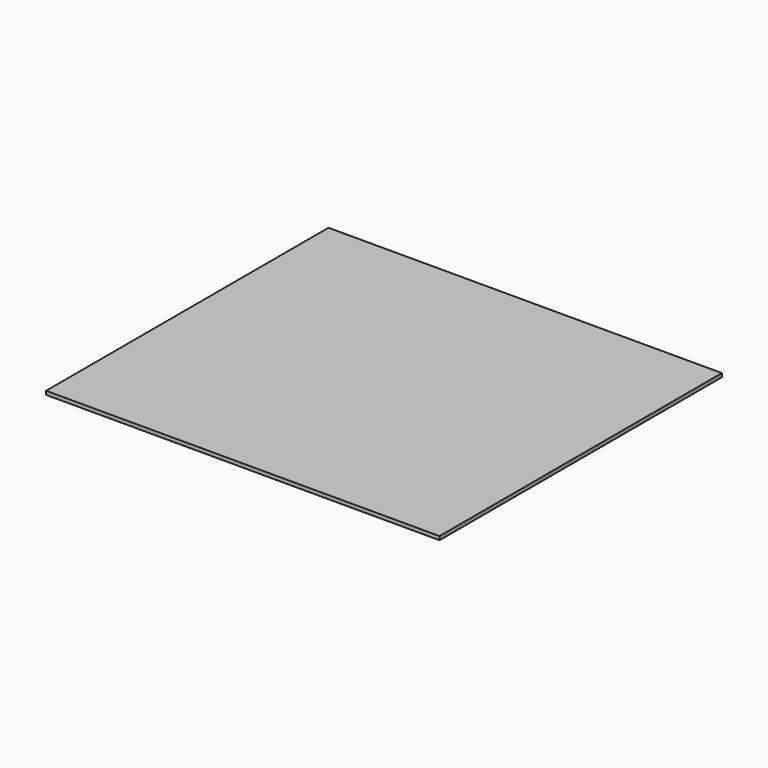
from build123d import *

# Parameters (mm, degrees)
F0_W     = 1358.9
F0_H     = 1219.2
F1_DEPTH = 12.7


# Not quite as in the source:
# - a feature names something its author has since deleted; it is built from what else it names


with BuildPart() as f1:
    # F0 (on Top) → F1 (new body)
    with BuildSketch(Plane.XY):
        with Locations((679.45, 609.6)):
            Rectangle(F0_W, F0_H)
    extrude(amount=F1_DEPTH)


solid = f1.part
